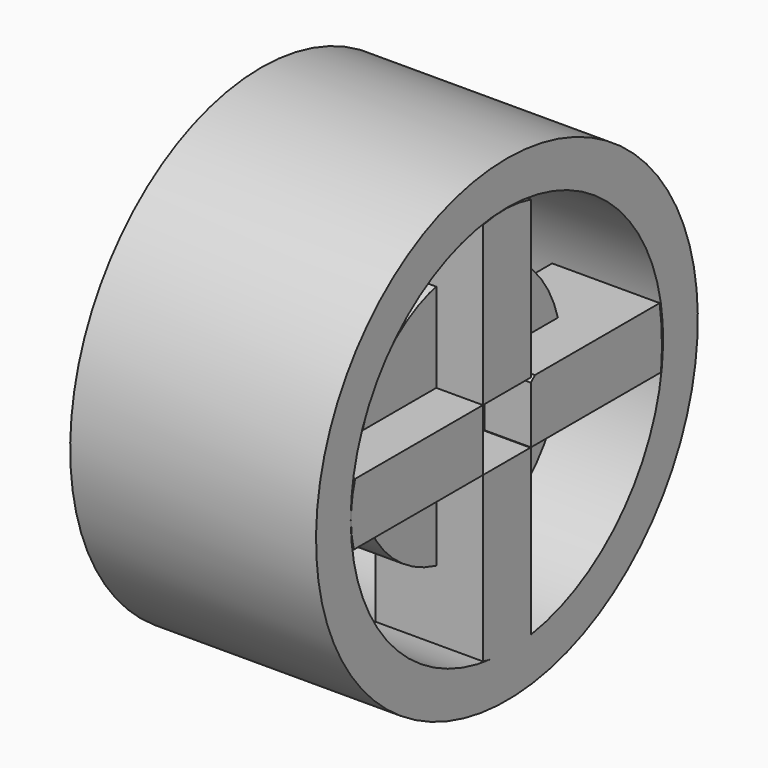
from build123d import *

# Parameters (mm, degrees)
F0_W     = 17
F0_H     = 3
F2_R     = 2.10545285
F3_DEPTH = 17.001
F5_DEPTH = 7.4320044443


# Not quite as in the source:
# - a feature of the source that left no trace in its solid (it failed there, or was rolled back) is left out


with BuildPart() as f1:
    # F0 (on Front) → F1 (revolve)
    with BuildSketch(Plane.XZ):
        Polygon((0, 4.3456270359), (0, 0), (13.7743903324, 0), (13.7743903324, 8.752326481), (9.5679955557, 8.752326481), (9.5679955557, 4.3456270359), align=None)
    revolve(axis=Axis((-17.2238798179, 0, 0), (1, 0, 0)))

    # F2 (on Right) → F3 (cut, through all)
    with BuildSketch(Plane.YZ):
        Circle(F2_R)
    extrude(amount=F3_DEPTH, mode=Mode.SUBTRACT)



with BuildPart() as f1b:
    # F0 (on Front) → F1, piece 2 (revolve)
    with BuildSketch(Plane.XZ):
        with Locations((8.5, 15)):
            Rectangle(F0_W, F0_H)
    revolve(axis=Axis((-17.2238798179, 0, 0), (1, 0, 0)))


with BuildPart() as f5:
    # F4 (on face) → F5 (new body, through all)
    with BuildSketch(Plane.YZ.offset(17)):
        with BuildLine():
            Line((2.075988996, 2.3240637966), (2.075988996, 3.8176883089))
            Line((2.075988996, 3.8176883089), (2.075988996, 13.1538297552))
            ThreePointArc((2.075988996, 13.1538297552), (0.0077885172, 13.4710626416), (-2.075988996, 13.2814282551))
            Line((-2.075988996, 13.2814282551), (-2.075988996, 3.8176883089))
            Line((-2.075988996, 3.8176883089), (-2.075988996, 2.3240637966))
            Line((-2.075988996, 2.3240637966), (2.075988996, 2.3240637966))
        make_face()
    extrude(amount=-F5_DEPTH)


with BuildPart() as f1_1:
    add(f1.part)

    add(f1b.part)  # F5#2 merges F1b
    # F4 (on face) → F5, piece 2 (join, through all)
    with BuildSketch(Plane.YZ.offset(17)):
        with BuildLine():
            Line((-2.075988996, -1.9356221886), (-2.075988996, 2.3240637966))
            Line((-2.075988996, 2.3240637966), (-13.1198950112, 2.3240637966))
            ThreePointArc((-13.1198950112, 2.3240637966), (-13.4767107858, 0.2025324211), (-13.2389972203, -1.9356221886))
            Line((-13.2389972203, -1.9356221886), (-3.8907378578, -1.9356221886))
            Line((-3.8907378578, -1.9356221886), (-2.075988996, -1.9356221886))
        make_face()
        with BuildLine():
            Line((2.41431853, 2.3240637966), (2.075988996, 1.9983820725))
            Line((2.075988996, 1.9983820725), (2.075988996, -1.9356221886))
            Line((2.075988996, -1.9356221886), (13.3207021949, -1.9356221886))
            ThreePointArc((13.3207021949, -1.9356221886), (13.3933684368, 0.1979176461), (13.2015999407, 2.3240637966))
            Line((13.2015999407, 2.3240637966), (2.41431853, 2.3240637966))
        make_face()
        with BuildLine():
            Line((2.075988996, -13.3378216997), (2.075988996, -1.9891557531))
            Line((2.075988996, -1.9891557531), (2.0244566825, -1.9356221886))
            Line((2.0244566825, -1.9356221886), (-2.0107918397, -1.9356221886))
            Line((-2.0107918397, -1.9356221886), (-2.075988996, -1.9983820725))
            Line((-2.075988996, -1.9983820725), (-2.075988996, -13.2782710716))
            ThreePointArc((-2.075988996, -13.2782710716), (-1.6646206015, -13.3695995078), (-1.2495113457, -13.4420504908))
            ThreePointArc((-1.2495113457, -13.4420504908), (0.4028347053, -13.4939884467), (2.049140015, -13.3435761773))
            ThreePointArc((2.049140015, -13.3435761773), (2.0625666461, -13.3407089263), (2.075988996, -13.3378216997))
        make_face()
    extrude(amount=-F5_DEPTH)


solid = Compound([f5.part, f1_1.part])
